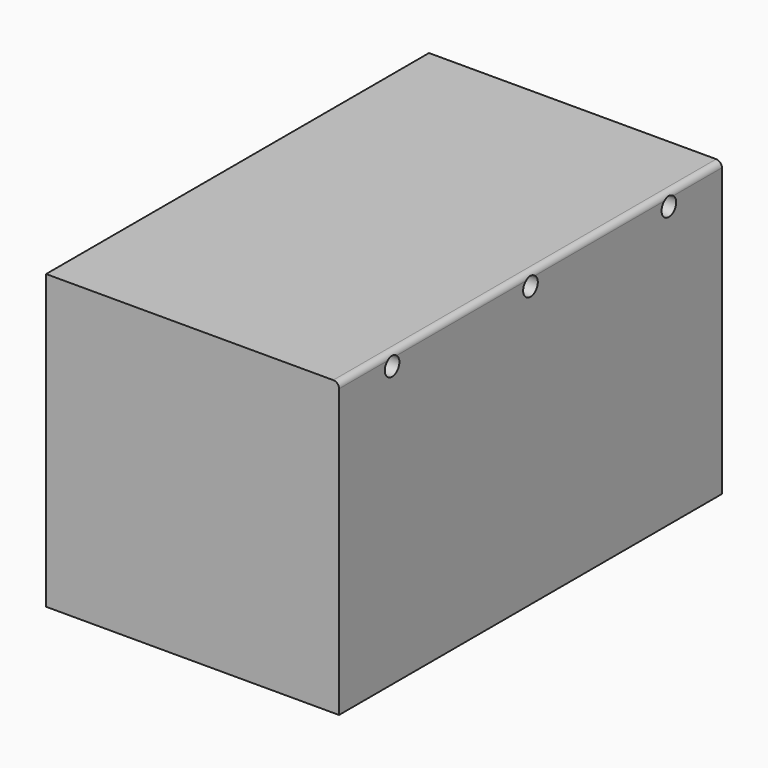
from build123d import *

# Parameters (mm, degrees)
F0_W        = 101.6
F0_H        = 101.6
F1_DEPTH    = 166
F2_R        = 3.175
F3_DEPTH    = 101.601
F4_T1_DEPTH = 176


# Not quite as in the source:
# - a fillet or chamfer that OpenCascade refuses, or shapes differently, is made with other operations: its cross-section is extruded or revolved along the edge and cut away or added


with BuildPart() as f1:
    # F0 (on Front) → F1 (new body)
    with BuildSketch(Plane.XZ):
        Rectangle(F0_W, F0_H)
    extrude(amount=F1_DEPTH)

    # F2 (on face) → F3 (cut, through all)
    with BuildSketch(Plane.YZ.offset(50.8)):
        with Locations((-143, 46.3)):
            Circle(F2_R)
        with Locations((-83, 46.3)):
            Circle(F2_R)
        with Locations((-23, 46.3)):
            Circle(F2_R)
    extrude(amount=-F3_DEPTH, mode=Mode.SUBTRACT)

    # F4: fillet of radius 2 on 1 edges, made by hand

    # F4_s2 → F4_t1 (cut)
    with BuildSketch(Plane.XZ.offset(-5)):
        with BuildLine():
            ThreePointArc((50.8, 48.8), (50.2142135624, 50.2142135624), (48.8, 50.8))
            Line((48.8, 50.8), (50.8, 50.8))
            Line((50.8, 50.8), (50.8, 48.8))
        make_face()
    extrude(amount=F4_T1_DEPTH, mode=Mode.SUBTRACT)


solid = f1.part
